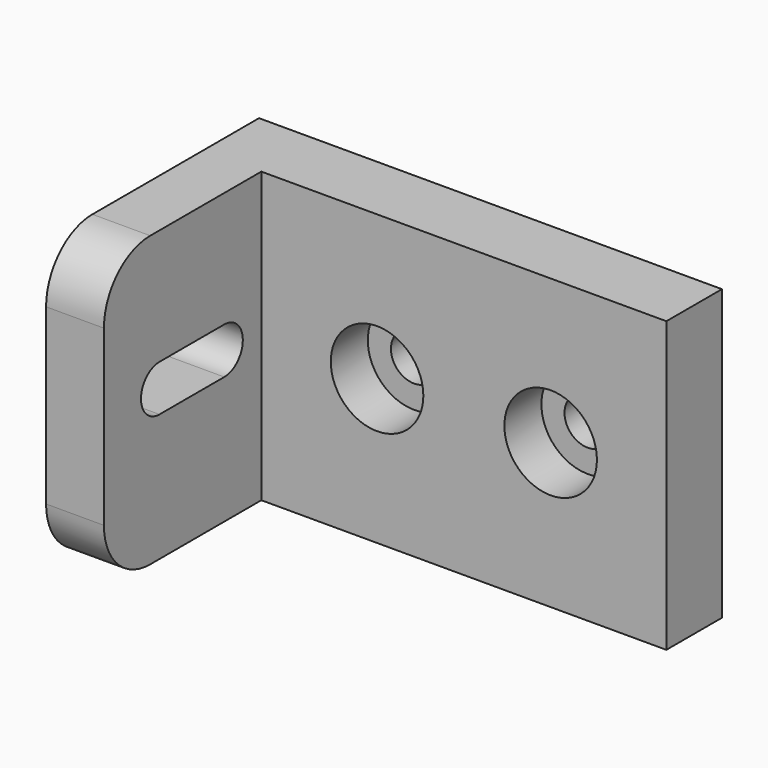
from build123d import *

# Parameters (mm, degrees)
F1_DEPTH       = 25
F2_R           = 5
F4_DEPTH       = 5.001
F6_D           = 4
F6_CBORE_D     = 8
F6_CBORE_DEPTH = 4


# Not quite as in the source:
# - a feature names something its author has since deleted; it is built from what else it names


with BuildPart() as f1:
    # F0 (on Top) → F1 (new body)
    with BuildSketch(Plane.XY):
        Polygon((0, 0), (0, -23), (5, -23), (5, -6), (40, -6), (40, 0), align=None)
    extrude(amount=F1_DEPTH)

    # F2
    f2_edges = [f1.edges().sort_by_distance(p)[0] for p in [
        (2.5, -23, 0),
        (2.5, -23, 25),
    ]]
    fillet(f2_edges, radius=F2_R)

    # F3 (on face) → F4 (cut, through all)
    with BuildSketch(Plane.YZ.offset(5)):
        with BuildLine():
            ThreePointArc((-17, 15), (-19, 13), (-17, 11))
            Line((-17, 11), (-10, 11))
            ThreePointArc((-10, 11), (-8, 13), (-10, 15))
            Line((-10, 15), (-17, 15))
        make_face()
    extrude(amount=-F4_DEPTH, mode=Mode.SUBTRACT)

    # F6 (through all)
    with Locations(Plane.XZ.offset(6)):
        with Locations((30, 12.5), (15, 12.5)):
            CounterBoreHole(F6_D / 2, F6_CBORE_D / 2, F6_CBORE_DEPTH)


solid = f1.part
